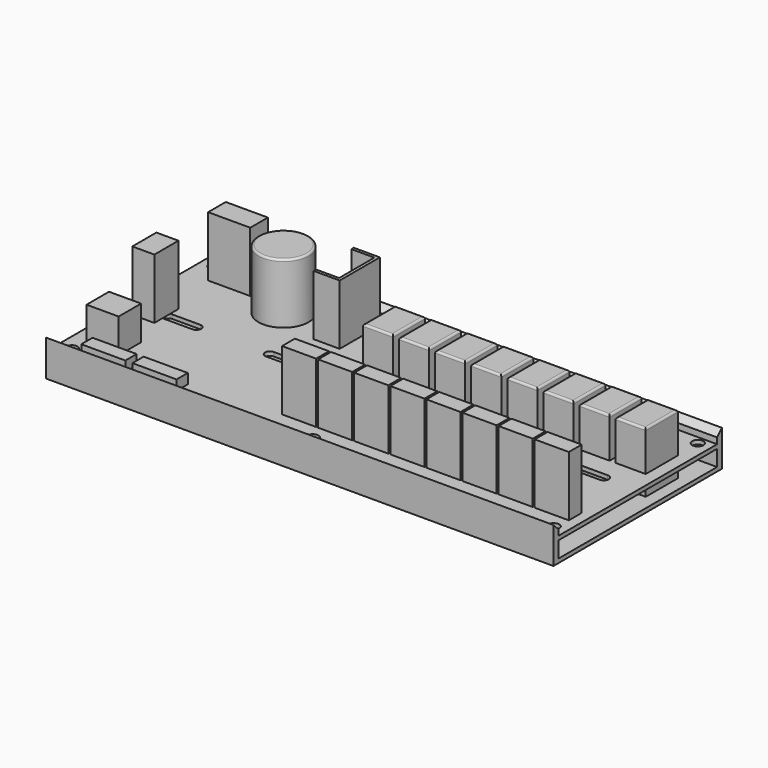
from build123d import *

# Parameters (mm, degrees)
F0_W      = 15
F0_H      = 20
F1_DEPTH  = 32
F0_W_2    = 253
F0_H_2    = 105
F0_W_3    = 17
F0_H_3    = 8
F2_DEPTH  = 12
F3_DEPTH  = 42
F4_W      = 253
F4_H      = 3
F5_DEPTH  = 6
F6_SIZE   = 2.99999
F7_W      = 11
F7_H      = 15
F7_W_2    = 21
F7_H_2    = 11
F7_R      = 12.5
F8_DEPTH  = 30
F9_R      = 1
F9_2_R    = 1
F9_3_R    = 1
F9_4_R    = 1
F9_5_R    = 1
F9_6_R    = 1
F9_7_R    = 1
F9_8_R    = 1
F9_9_R    = 1
F10_W     = 16
F10_H     = 14
F11_DEPTH = 17
F12_W     = 22
F12_H     = 7
F13_DEPTH = 5
F15_DEPTH = 12.001
F14_R     = 2.8
F16_DEPTH = 9
F17_W     = 99
F17_H     = 8
F18_DEPTH = 253.001


# Not quite as in the source:
# - a fillet or chamfer is up to 0.001 mm smaller than in the source, because OpenCascade refuses the exact size


with BuildPart() as f1:
    # F0 (on Top) → F1 (new body)
    with BuildSketch(Plane.XY):
        with Locations((-13, 22.5)):
            Rectangle(F0_W, F0_H)
    extrude(amount=F1_DEPTH)

    # F9
    f9_edges = [f1.edges().sort_by_distance(p)[0] for p in [
        (-13, 32.5, 32),
        (-20.5, 22.5, 32),
        (-13, 12.5, 32),
        (-5.5, 22.5, 32),
    ]]
    fillet(f9_edges, radius=F9_R)


with BuildPart() as f1b:
    # F0 (on Top) → F1, piece 2 (new body)
    with BuildSketch(Plane.XY):
        with Locations((5, 22.5)):
            Rectangle(F0_W, F0_H)
    extrude(amount=F1_DEPTH)

    # F9#2
    f9_2_edges = [f1b.edges().sort_by_distance(p)[0] for p in [
        (5, 32.5, 32),
        (-2.5, 22.5, 32),
        (5, 12.5, 32),
        (12.5, 22.5, 32),
    ]]
    fillet(f9_2_edges, radius=F9_2_R)


with BuildPart() as f1c:
    # F0 (on Top) → F1, piece 3 (new body)
    with BuildSketch(Plane.XY):
        with Locations((23, 22.5)):
            Rectangle(F0_W, F0_H)
    extrude(amount=F1_DEPTH)

    # F9#3
    f9_3_edges = [f1c.edges().sort_by_distance(p)[0] for p in [
        (23, 32.5, 32),
        (15.5, 22.5, 32),
        (23, 12.5, 32),
        (30.5, 22.5, 32),
    ]]
    fillet(f9_3_edges, radius=F9_3_R)


with BuildPart() as f1d:
    # F0 (on Top) → F1, piece 4 (new body)
    with BuildSketch(Plane.XY):
        with Locations((41, 22.5)):
            Rectangle(F0_W, F0_H)
    extrude(amount=F1_DEPTH)

    # F9#4
    f9_4_edges = [f1d.edges().sort_by_distance(p)[0] for p in [
        (41, 32.5, 32),
        (33.5, 22.5, 32),
        (41, 12.5, 32),
        (48.5, 22.5, 32),
    ]]
    fillet(f9_4_edges, radius=F9_4_R)


with BuildPart() as f1e:
    # F0 (on Top) → F1, piece 5 (new body)
    with BuildSketch(Plane.XY):
        with Locations((59, 22.5)):
            Rectangle(F0_W, F0_H)
    extrude(amount=F1_DEPTH)

    # F9#5
    f9_5_edges = [f1e.edges().sort_by_distance(p)[0] for p in [
        (59, 32.5, 32),
        (51.5, 22.5, 32),
        (59, 12.5, 32),
        (66.5, 22.5, 32),
    ]]
    fillet(f9_5_edges, radius=F9_5_R)


with BuildPart() as f1f:
    # F0 (on Top) → F1, piece 6 (new body)
    with BuildSketch(Plane.XY):
        with Locations((77, 22.5)):
            Rectangle(F0_W, F0_H)
    extrude(amount=F1_DEPTH)

    # F9#6
    f9_6_edges = [f1f.edges().sort_by_distance(p)[0] for p in [
        (77, 32.5, 32),
        (69.5, 22.5, 32),
        (77, 12.5, 32),
        (84.5, 22.5, 32),
    ]]
    fillet(f9_6_edges, radius=F9_6_R)


with BuildPart() as f1g:
    # F0 (on Top) → F1, piece 7 (new body)
    with BuildSketch(Plane.XY):
        with Locations((95, 22.5)):
            Rectangle(F0_W, F0_H)
    extrude(amount=F1_DEPTH)

    # F9#7
    f9_7_edges = [f1g.edges().sort_by_distance(p)[0] for p in [
        (95, 32.5, 32),
        (87.5, 22.5, 32),
        (95, 12.5, 32),
        (102.5, 22.5, 32),
    ]]
    fillet(f9_7_edges, radius=F9_7_R)


with BuildPart() as f1h:
    # F0 (on Top) → F1, piece 8 (new body)
    with BuildSketch(Plane.XY):
        with Locations((113, 22.5)):
            Rectangle(F0_W, F0_H)
    extrude(amount=F1_DEPTH)

    # F9#8
    f9_8_edges = [f1h.edges().sort_by_distance(p)[0] for p in [
        (113, 32.5, 32),
        (105.5, 22.5, 32),
        (113, 12.5, 32),
        (120.5, 22.5, 32),
    ]]
    fillet(f9_8_edges, radius=F9_8_R)


with BuildPart() as f2:
    # F0 (on Top) → F2 (new body)
    with BuildSketch(Plane.XY):
        Rectangle(F0_W_2, F0_H_2)
        with Locations((-13, -32.6770811379)):
            Rectangle(F0_W_3, F0_H_3, mode=Mode.SUBTRACT)
        with Locations((5, -32.6770811379)):
            Rectangle(F0_W_3, F0_H_3, mode=Mode.SUBTRACT)
        with Locations((23, -32.6770811379)):
            Rectangle(F0_W_3, F0_H_3, mode=Mode.SUBTRACT)
        with Locations((41, -32.6770811379)):
            Rectangle(F0_W_3, F0_H_3, mode=Mode.SUBTRACT)
        with Locations((59, -32.6770811379)):
            Rectangle(F0_W_3, F0_H_3, mode=Mode.SUBTRACT)
        with Locations((77, -32.6770811379)):
            Rectangle(F0_W_3, F0_H_3, mode=Mode.SUBTRACT)
        with Locations((95, -32.6770811379)):
            Rectangle(F0_W_3, F0_H_3, mode=Mode.SUBTRACT)
        with Locations((113, -32.6770811379)):
            Rectangle(F0_W_3, F0_H_3, mode=Mode.SUBTRACT)
        with Locations((-13, 22.5)):
            Rectangle(F0_W, F0_H, mode=Mode.SUBTRACT)
        with Locations((5, 22.5)):
            Rectangle(F0_W, F0_H, mode=Mode.SUBTRACT)
        with Locations((23, 22.5)):
            Rectangle(F0_W, F0_H, mode=Mode.SUBTRACT)
        with Locations((41, 22.5)):
            Rectangle(F0_W, F0_H, mode=Mode.SUBTRACT)
        with Locations((59, 22.5)):
            Rectangle(F0_W, F0_H, mode=Mode.SUBTRACT)
        with Locations((77, 22.5)):
            Rectangle(F0_W, F0_H, mode=Mode.SUBTRACT)
        with Locations((95, 22.5)):
            Rectangle(F0_W, F0_H, mode=Mode.SUBTRACT)
        with Locations((113, 22.5)):
            Rectangle(F0_W, F0_H, mode=Mode.SUBTRACT)
    extrude(amount=F2_DEPTH)

    # F0 (on Top) → F3 (join)
    with BuildSketch(Plane.XY):
        with Locations((-13, -32.6770811379)):
            Rectangle(F0_W_3, F0_H_3)
        with Locations((5, -32.6770811379)):
            Rectangle(F0_W_3, F0_H_3)
        with Locations((23, -32.6770811379)):
            Rectangle(F0_W_3, F0_H_3)
        with Locations((41, -32.6770811379)):
            Rectangle(F0_W_3, F0_H_3)
        with Locations((59, -32.6770811379)):
            Rectangle(F0_W_3, F0_H_3)
        with Locations((77, -32.6770811379)):
            Rectangle(F0_W_3, F0_H_3)
        with Locations((95, -32.6770811379)):
            Rectangle(F0_W_3, F0_H_3)
        with Locations((113, -32.6770811379)):
            Rectangle(F0_W_3, F0_H_3)
    extrude(amount=F3_DEPTH)

    # F4 (on face) → F5 (join)
    with BuildSketch(Plane.XY.offset(12)):
        with Locations((0, 51)):
            Rectangle(F4_W, F4_H)
        with Locations((0, -51)):
            Rectangle(F4_W, F4_H)
    extrude(amount=F5_DEPTH)

    # F6 (size 3 in the source; OpenCascade refuses exactly that, so slightly less here)
    f6_edges = [f2.edges().sort_by_distance(p)[0] for p in [
        (0, 49.5, 18),
        (0, -49.5, 18),
    ]]
    chamfer(f6_edges, length=F6_SIZE)

    # F7 (on face) → F8 (join)
    with BuildSketch(Plane.XY.offset(12)):
        with Locations((-114, 0)):
            Rectangle(F7_W, F7_H)
        with Locations((-104, 39)):
            Rectangle(F7_W_2, F7_H_2)
        with Locations((-74.5, 30.5)):
            Circle(F7_R)
        Polygon((-38.5, 45.5), (-51.5, 45.5), (-51.5, 44), (-40, 44), (-40, 22), (-51.5, 22), (-51.5, 20.5), (-38.5, 20.5), align=None)
    extrude(amount=F8_DEPTH)

    # F9#9
    f9_9_edges = [f2.edges().sort_by_distance(p)[0] for p in [
        (-87, 30.5, 42),
    ]]
    fillet(f9_9_edges, radius=F9_9_R)

    # F10 (on face) → F11 (join)
    with BuildSketch(Plane.XY.offset(12)):
        with Locations((-110.3310795426, -30.4876260757)):
            Rectangle(F10_W, F10_H)
    extrude(amount=F11_DEPTH)

    # F12 (on face) → F13 (join)
    with BuildSketch(Plane.XY.offset(12)):
        with Locations((-102.5, -43.3088723719)):
            Rectangle(F12_W, F12_H)
        with Locations((-77, -43.3088723719)):
            Rectangle(F12_W, F12_H)
    extrude(amount=F13_DEPTH)

    # F14 (on face) → F15 (cut, through all)
    with BuildSketch(Plane.XY.offset(12)):
        with BuildLine():
            ThreePointArc((-56.8500881126, 2.450439948), (-59.300029372, 0.0003812091), (-56.8499706331, -2.4495600502))
            Line((-56.8499706331, -2.4495600502), (-42.750000007, -2.4492219978))
            ThreePointArc((-42.750000007, -2.4492219978), (-40.3001012629, 0.0152115547), (-42.7788666164, 2.4506086297))
            Line((-42.7788666164, 2.4506086297), (-56.8500881126, 2.450439948))
        make_face()
        with BuildLine():
            ThreePointArc((8.0506018618, -2.4472260314), (10.5004415194, 0.0172662576), (8.0216177771, 2.4526039025))
            Line((8.0216177771, 2.4526039025), (-6.049603711, 2.4520978578))
            ThreePointArc((-6.049603711, 2.4520978578), (-8.4994862286, 0.0019803814), (-6.0493687521, -2.4479021362))
            Line((-6.0493687521, -2.4479021362), (8.0506018618, -2.4472260314))
        make_face()
        with BuildLine():
            Line((44.7223665114, -2.4460762204), (58.8223371254, -2.4454001156))
            ThreePointArc((58.8223371254, -2.4454001156), (61.2722196429, 0.0047173608), (58.8221021665, 2.4545998784))
            Line((58.8221021665, 2.4545998784), (44.7508806945, 2.4537564706))
            ThreePointArc((44.7508806945, 2.4537564706), (42.2722905163, 0.0181811137), (44.7223665114, -2.4460762204))
        make_face()
        with BuildLine():
            ThreePointArc((95.5220433605, 2.4567996174), (93.0722195862, 0.0066234048), (95.5223957988, -2.4432003696))
            Line((95.5223957988, -2.4432003696), (109.6223663925, -2.4421862125))
            ThreePointArc((109.6223663925, -2.4421862125), (112.0721469622, 0.0223648117), (109.5932648324, 2.4576430252))
            Line((109.5932648324, 2.4576430252), (95.5220433605, 2.4567996174))
        make_face()
        with BuildLine():
            Line((-93.5500293699, 2.4499999998), (-107.6212508661, 2.4498313181))
            ThreePointArc((-107.6212508661, 2.4498313181), (-108.0675999545, 2.4141479404), (-108.5, 2.2978250586))
            Line((-108.5, 2.2978250586), (-108.5, -2.2978250586))
            ThreePointArc((-108.5, -2.2978250586), (-108.0817572272, -2.4116562145), (-107.65, -2.45))
            Line((-107.65, -2.45), (-93.5500293698, -2.4499999998))
            ThreePointArc((-93.5500293698, -2.4499999998), (-91.10002937, 0), (-93.5500293699, 2.4499999998))
        make_face()
        with BuildLine():
            Line((-108.5, -2.2978250586), (-108.5, 2.2978250586))
            ThreePointArc((-108.5, 2.2978250586), (-110.1, 0), (-108.5, -2.2978250586))
        make_face()
    extrude(amount=-F15_DEPTH, mode=Mode.SUBTRACT)

    # F14 (on face) → F16 (cut)
    with BuildSketch(Plane.XY.offset(12)):
        with Locations((-120.1, 44.4)):
            Circle(F14_R)
        with Locations((0, 45.5)):
            Circle(F14_R)
        with Locations((120.1, 45.5)):
            Circle(F14_R)
        with Locations((120.1, -44.4)):
            Circle(F14_R)
        with Locations((0, -44.4)):
            Circle(F14_R)
        with Locations((-120.1, -44.4)):
            Circle(F14_R)
    extrude(amount=-F16_DEPTH, mode=Mode.SUBTRACT)

    # F17 (on face) → F18 (cut, through all)
    with BuildSketch(Plane(origin=(-126.5, 0, 0), x_dir=(0, -1, 0), z_dir=(-1, 0, 0))):
        with Locations((0, 6)):
            Rectangle(F17_W, F17_H)
    extrude(amount=-F18_DEPTH, mode=Mode.SUBTRACT)


solid = Compound([f1.part, f1b.part, f1c.part, f1d.part, f1e.part, f1f.part, f1g.part, f1h.part, f2.part])
